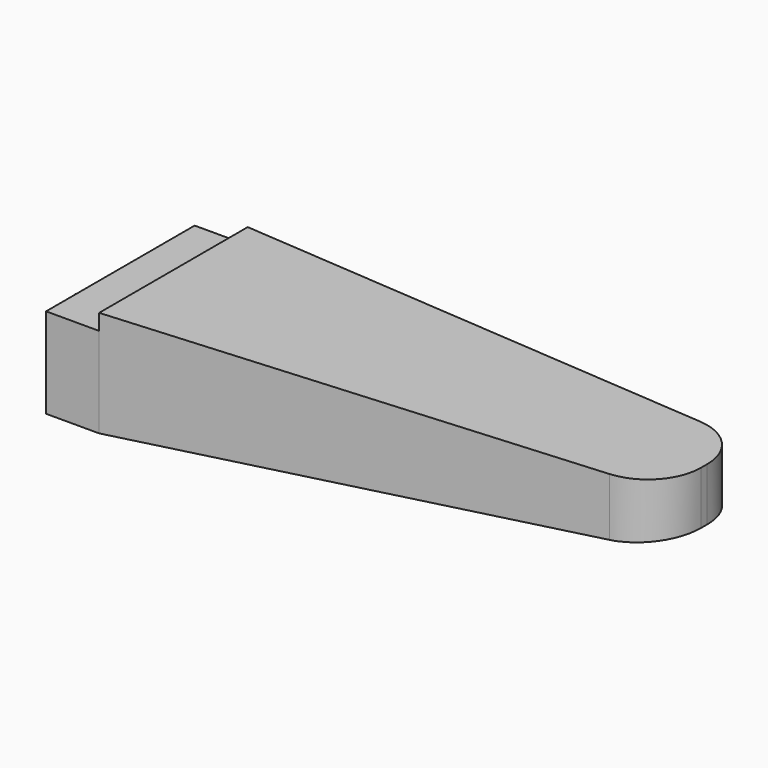
from build123d import *

# Parameters (mm, degrees)
F1_DEPTH = 10
F2_DEPTH = 17
F3_W     = 100
F3_H     = 35
F4_DEPTH = 3
F5_SIZE2 = 10
F5_SIZE  = 100
F6_SIZE2 = 99.99999
F6_SIZE  = 7.49999
F7_R     = 10


# Not quite as in the source:
# - a fillet or chamfer is up to 0.001 mm smaller than in the source, because OpenCascade refuses the exact size


with BuildPart() as f1:
    # F0 (on Top) → F1 (new body)
    with BuildSketch(Plane.XY):
        Polygon((-58.5, -8.5), (-58.5, -2.5), (-58.5, 0), (-58.5, 2.5), (-58.5, 8.5), (-63.5, 0), align=None)
        Polygon((-58.5, -2.5), (-55, -2.5), (-55, 2.5), (-58.5, 2.5), (-58.5, 0), align=None)
    extrude(amount=F1_DEPTH)

    # F0 (on Top) → F2 (join)
    with BuildSketch(Plane.XY):
        Polygon((-55, -17.5), (55, -17.5), (55, 17.5), (-55, 17.5), (-55, 2.5), (-55, -2.5), align=None)
    extrude(amount=F2_DEPTH)

    # F3 (on face) → F4 (join)
    with BuildSketch(Plane.XY.offset(17)):
        with Locations((5, 0)):
            Rectangle(F3_W, F3_H)
    extrude(amount=F4_DEPTH)

    # F5
    f5_edges = [f1.edges().sort_by_distance(p)[0] for p in [
        (55, 0, 0),
    ]]
    f5_side = f1.faces().sort_by_distance((-0.907982, 0, 0))[0]
    chamfer(f5_edges, length=F5_SIZE, length2=F5_SIZE2, reference=f5_side)

    # F6 (size 7.5 and 100 in the source; OpenCascade refuses exactly that, so slightly less here)
    f6_edges = [f1.edges().sort_by_distance(p)[0] for p in [
        (55, -17.5, 15),
        (55, 17.5, 15),
    ]]
    f6_side = f1.faces().sort_by_distance((55, 0, 15))[0]
    chamfer(f6_edges, length=F6_SIZE, length2=F6_SIZE2, reference=f6_side)

    # F7
    f7_edges = [f1.edges().sort_by_distance(p)[0] for p in [
        (55, -10.00001, 15),
        (55, 10.00001, 15),
    ]]
    fillet(f7_edges, radius=F7_R)


solid = f1.part
